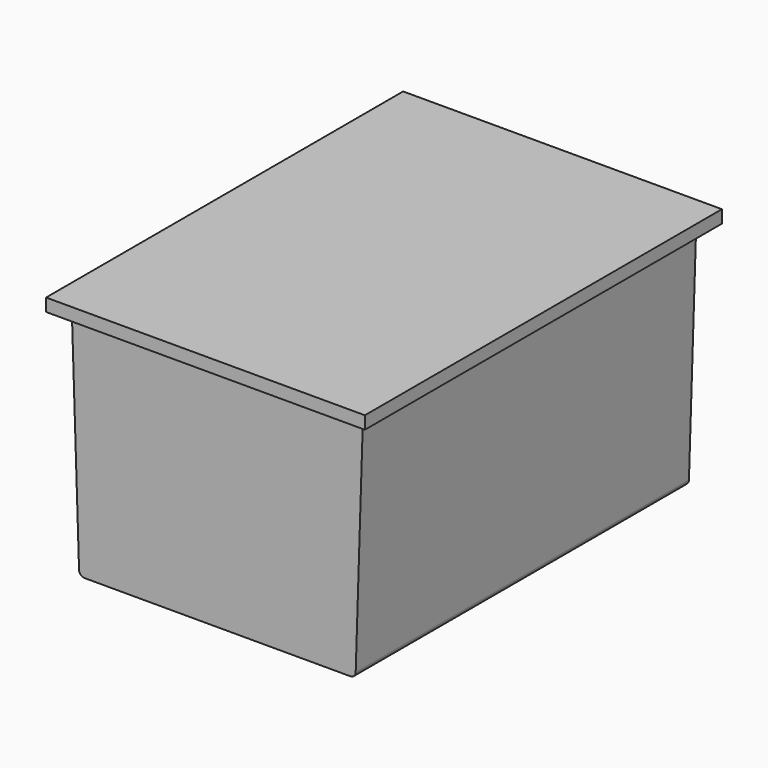
from build123d import *

# Parameters (mm, degrees)
F1_DEPTH = 420
F3_DEPTH = 14


# Not quite as in the source:
# - a pattern or mirror of a feature is missing from the dataset's text; its kind, count and spacing are read off the source's solid


with BuildPart() as f1:
    # F0 (on Front) → F1 (new body)
    with BuildSketch(Plane.XZ):
        with BuildLine():
            Line((150, 0), (0, 0))
            Line((0, 0), (-150, 0))
            Line((-150, 0), (-150, -12))
            Line((-150, -12), (-141.8420265222, -12))
            ThreePointArc((-141.8420265222, -12), (-138.3636891874, -13.4081802125), (-136.8446021756, -16.8395322458))
            Line((-136.8446021756, -16.8395322458), (-130.1553978244, -225.1604677542))
            ThreePointArc((-130.1553978244, -225.1604677542), (-128.6363108126, -228.5918197875), (-125.1579734778, -230))
            Line((-125.1579734778, -230), (0, -230))
            Line((0, -230), (125.1579734778, -230))
            ThreePointArc((125.1579734778, -230), (128.6363108126, -228.5918197875), (130.1553978244, -225.1604677542))
            Line((130.1553978244, -225.1604677542), (136.8446021756, -16.8395322458))
            ThreePointArc((136.8446021756, -16.8395322458), (138.3636891874, -13.4081802125), (141.8420265222, -12))
            Line((141.8420265222, -12), (150, -12))
            Line((150, -12), (150, 0))
        make_face()
    extrude(amount=F1_DEPTH)

    # F2 (on face) → F3 (cut)
    with BuildSketch(Plane.XZ.offset(420)):
        with BuildLine():
            Line((141.8420265222, -12), (-141.8420265222, -12))
            ThreePointArc((-141.8420265222, -12), (-138.3636891874, -13.4081802125), (-136.8446021756, -16.8395322458))
            Line((-136.8446021756, -16.8395322458), (-130.1553978244, -225.1604677542))
            ThreePointArc((-130.1553978244, -225.1604677542), (-128.6363108126, -228.5918197875), (-125.1579734778, -230))
            Line((-125.1579734778, -230), (125.1579734778, -230))
            ThreePointArc((125.1579734778, -230), (128.6363108126, -228.5918197875), (130.1553978244, -225.1604677542))
            Line((130.1553978244, -225.1604677542), (136.8446021756, -16.8395322458))
            ThreePointArc((136.8446021756, -16.8395322458), (138.3636891874, -13.4081802125), (141.8420265222, -12))
        make_face()
    f3 = extrude(amount=-F3_DEPTH, mode=Mode.SUBTRACT)

    # F3_copies: F3 across plane
    add(f3.mirror(Plane.ZX.offset(-210)), mode=Mode.SUBTRACT)


solid = f1.part
